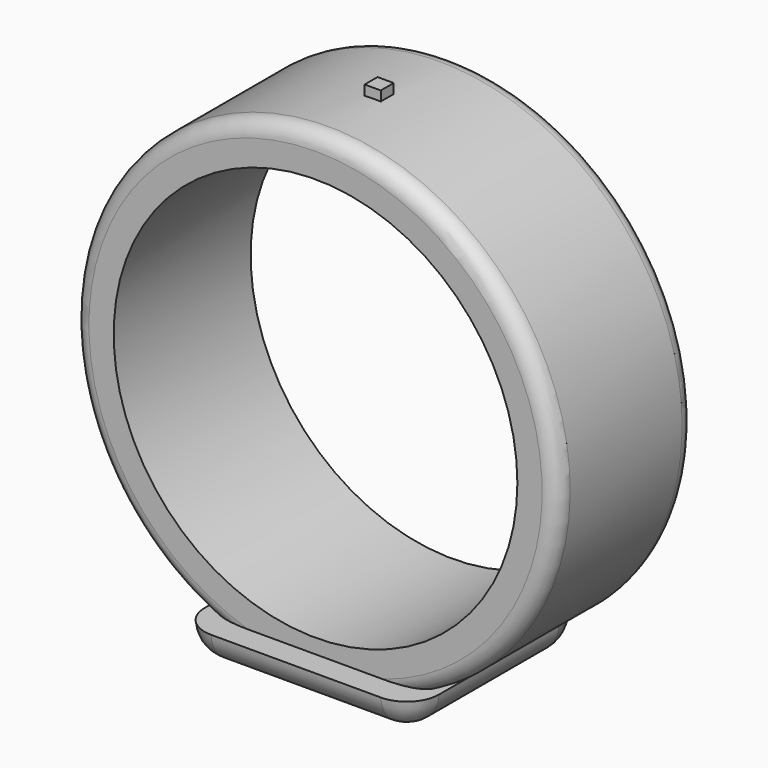
from build123d import *

# Parameters (mm, degrees)
F0_R         = 38.1
F0_R_2       = 31.75
F1_DEPTH     = 26.924
F2_R         = 2.4528409794
F4_START     = -34.036
F3_W         = 36.8709713221
F3_H         = 33.7369362824
F4_DEPTH     = 4.826
F5_R         = 5.08
F6_W         = 26.7109713221
F6_H         = 23.5769362824
F7_DEPTH     = 4.826
F8_T1_DEPTH  = 26.7109713221
F8_T3_DEPTH  = 23.5769362824
F8_T6_ANGLE  = 90
F8_T8_ANGLE  = 90
F8_T10_ANGLE = 90
F8_T12_ANGLE = 90
F9_W         = 6.8778875601
F9_H         = 2.9623268638
F10_DEPTH    = 4.8006
F12_START    = 31.75
F11_W        = 2.54
F11_H        = 2.54
F12_DEPTH    = 7.874


# Not quite as in the source:
# - a fillet or chamfer that OpenCascade refuses, or shapes differently, is made with other operations: its cross-section is extruded or revolved along the edge and cut away or added


with BuildPart() as f1:
    # F0 (on Front) → F1 (new body)
    with BuildSketch(Plane.XZ):
        Circle(F0_R)
        Circle(F0_R_2, mode=Mode.SUBTRACT)
    extrude(amount=F1_DEPTH)

    # F2
    f2_edges = [f1.edges().sort_by_distance(p)[0] for p in [
        (-38.1, -26.924, 0),
        (-38.1, 0, 0),
    ]]
    fillet(f2_edges, radius=F2_R)

    # F3 (on Top) → F4 (join)
    with BuildSketch(Plane.XY.offset(F4_START)):
        with Locations((0.0921785831, -14.0109679196)):
            Rectangle(F3_W, F3_H)
    extrude(amount=-F4_DEPTH)

    # F5
    f5_edges = [f1.edges().sort_by_distance(p)[0] for p in [
        (-18.343307, 2.8575, -36.449),
        (18.527664, 2.8575, -36.449),
        (18.527664, -30.879436, -36.449),
        (-18.343307, -30.879436, -36.449),
    ]]
    fillet(f5_edges, radius=F5_R)

    # F6 (on face) → F7 (cut)
    with BuildSketch(Plane(origin=(0, 0, -38.862), x_dir=(1, 0, 0), z_dir=(0, 0, -1))):
        with Locations((0.0921785831, 14.0109679196)):
            Rectangle(F6_W, F6_H)
    extrude(amount=-F7_DEPTH, mode=Mode.SUBTRACT)

    # F8: fillet of radius 5.08 on 1 edges, made by hand

    # F8_s2 → F8_t1 (cut)
    with BuildSketch(Plane.YZ.offset(-13.2633070779)):
        with BuildLine():
            ThreePointArc((-30.8794360608, -34.036), (-29.3069384175, -37.4628096935), (-25.8057900345, -38.862))
            Line((-25.8057900345, -38.862), (-30.8794360608, -38.862))
            Line((-30.8794360608, -38.862), (-30.8794360608, -34.036))
        make_face()
        with BuildLine():
            ThreePointArc((2.8575002216, -34.036), (1.2850025783, -37.4628096935), (-2.2161458047, -38.862))
            Line((-2.2161458047, -38.862), (2.8575002216, -38.862))
            Line((2.8575002216, -38.862), (2.8575002216, -34.036))
        make_face()
    extrude(amount=F8_T1_DEPTH, mode=Mode.SUBTRACT)

    # F8_s4 → F8_t3 (cut)
    with BuildSketch(Plane.XZ.offset(2.2224997784)):
        with BuildLine():
            ThreePointArc((18.5276642442, -34.036), (16.9551666009, -37.4628096935), (13.4540182179, -38.862))
            Line((13.4540182179, -38.862), (18.5276642442, -38.862))
            Line((18.5276642442, -38.862), (18.5276642442, -34.036))
        make_face()
        with BuildLine():
            ThreePointArc((-18.3433070779, -34.036), (-16.7708094346, -37.4628096935), (-13.2696610516, -38.862))
            Line((-13.2696610516, -38.862), (-18.3433070779, -38.862))
            Line((-18.3433070779, -38.862), (-18.3433070779, -34.036))
        make_face()
    extrude(amount=F8_T3_DEPTH, mode=Mode.SUBTRACT)

    # F8_s5 → F8_t6 (revolve, cut)
    with BuildSketch(Plane.YZ.offset(-13.2633070779)):
        with BuildLine():
            ThreePointArc((-30.8794360608, -34.036), (-29.3069384175, -37.4628096935), (-25.8057900345, -38.862))
            Line((-25.8057900345, -38.862), (-30.8794360608, -38.862))
            Line((-30.8794360608, -38.862), (-30.8794360608, -34.036))
        make_face()
    revolve(axis=Axis((-13.2633070779, -25.7994360608, -38.862), (0, 0, -1)), revolution_arc=F8_T6_ANGLE, mode=Mode.SUBTRACT)

    # F8_s7 → F8_t8 (revolve, cut)
    with BuildSketch(Plane.XZ.offset(25.7994360608)):
        with BuildLine():
            ThreePointArc((18.5276642442, -34.036), (16.9551666009, -37.4628096935), (13.4540182179, -38.862))
            Line((13.4540182179, -38.862), (18.5276642442, -38.862))
            Line((18.5276642442, -38.862), (18.5276642442, -34.036))
        make_face()
    revolve(axis=Axis((13.4476642442, -25.7994360608, -38.862), (0, 0, -1)), revolution_arc=F8_T8_ANGLE, mode=Mode.SUBTRACT)

    # F8_s9 → F8_t10 (revolve, cut)
    with BuildSketch(Plane.XZ.offset(2.2224997784)):
        with BuildLine():
            ThreePointArc((18.5276642442, -34.036), (16.9551666009, -37.4628096935), (13.4540182179, -38.862))
            Line((13.4540182179, -38.862), (18.5276642442, -38.862))
            Line((18.5276642442, -38.862), (18.5276642442, -34.036))
        make_face()
    revolve(axis=Axis((13.4476642442, -2.2224997784, -38.862), (0, 0, 1)), revolution_arc=F8_T10_ANGLE, mode=Mode.SUBTRACT)

    # F8_s11 → F8_t12 (revolve, cut)
    with BuildSketch(Plane.YZ.offset(-13.2633070779)):
        with BuildLine():
            ThreePointArc((2.8575002216, -34.036), (1.2850025783, -37.4628096935), (-2.2161458047, -38.862))
            Line((-2.2161458047, -38.862), (2.8575002216, -38.862))
            Line((2.8575002216, -38.862), (2.8575002216, -34.036))
        make_face()
    revolve(axis=Axis((-13.2633070779, -2.2224997784, -38.862), (0, 0, 1)), revolution_arc=F8_T12_ANGLE, mode=Mode.SUBTRACT)

    # F9 (on face) → F10 (join)
    with BuildSketch(Plane(origin=(0, 0, -34.036), x_dir=(1, 0, 0), z_dir=(0, 0, -1))):
        with Locations((-9.8243632978, 12.5298044877)):
            Rectangle(F9_W, F9_H)
    extrude(amount=F10_DEPTH)

    # F11 (on Top) → F12 (join)
    with BuildSketch(Plane.XY.offset(F12_START)):
        with Locations((-0.3243902236, -14.0109681524)):
            Rectangle(F11_W, F11_H)
    extrude(amount=F12_DEPTH)


solid = f1.part
